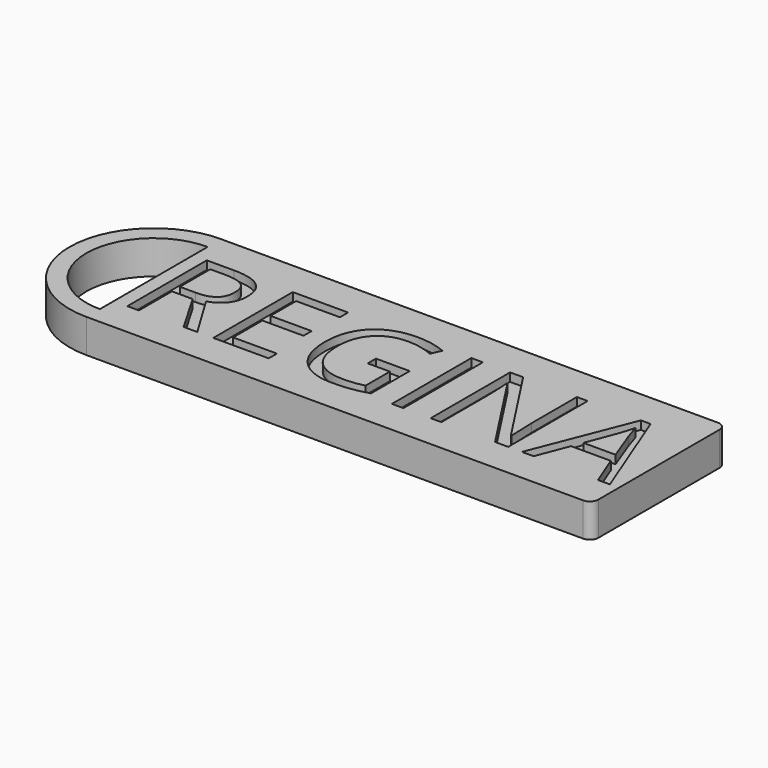
from build123d import *

# Parameters (mm, degrees)
F4_DEPTH     = 2
F1_TEXT_SIZE = 8.2587749484
F2_DEPTH     = 0.5
F3_R         = 0.5


# Not quite as in the source:
# - Text() gives the source's letters only with a copy of the font that has no kerning and outlines rounded to 1/6400 em; it was checked with that copy


with BuildPart() as f4:
    # F0 (on Top) → F4 (new body)
    with BuildSketch(Plane.XY):
        Polygon((24.7291392038, 3.2207785361), (-5.2708607962, 3.2207785361), (-5.2708607962, 2.2207785361), (-5.2708607962, -5.7792214639), (-5.2708607962, -6.7792214639), (24.7291392038, -6.7792214639), align=None)
        with BuildLine():
            Line((-5.2708607962, 2.2207785361), (-5.2708607962, 3.2207785361))
            ThreePointArc((-5.2708607962, 3.2207785361), (-10.2708607962, -1.7792214639), (-5.2708607962, -6.7792214639))
            Line((-5.2708607962, -6.7792214639), (-5.2708607962, -5.7792214639))
            ThreePointArc((-5.2708607962, -5.7792214639), (-9.2708607962, -1.7792214639), (-5.2708607962, 2.2207785361))
        make_face()
    extrude(amount=F4_DEPTH)

    # F1 (on face) → F2 (cut)
    with BuildSketch(Plane.XY.offset(2)):
        with Locations((-5.2708607962, -4.7523804454)):
            Text('REGINA', F1_TEXT_SIZE, font='Open Sans', text_align=(TextAlign.LEFT, TextAlign.BOTTOM))
    extrude(amount=-F2_DEPTH, mode=Mode.SUBTRACT)

    # F3
    f3_edges = [f4.edges().sort_by_distance(p)[0] for p in [
        (24.729139, -6.779221, 1),
        (24.729139, 3.220779, 1),
    ]]
    fillet(f3_edges, radius=F3_R)


solid = f4.part
